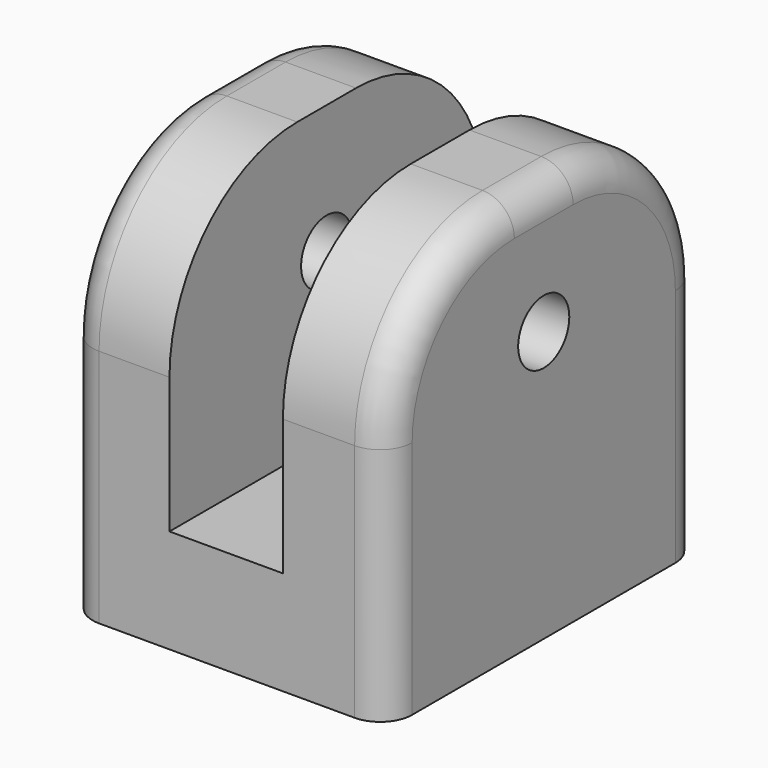
from build123d import *

# Parameters (mm, degrees)
F0_W     = 20
F0_H     = 24.5975396182
F1_DEPTH = 25
F2_W     = 7.1
F2_H     = 19.9254054902
F3_DEPTH = 12.5
F4_R     = 2
F5_DEPTH = 20.001
F6_R     = 10
F7_R     = 2
F8_R     = 2


with BuildPart() as f1:
    # F0 (on Top) → F1 (new body)
    with BuildSketch(Plane.XY):
        Rectangle(F0_W, F0_H)
    extrude(amount=F1_DEPTH)

    # F2 (on Front) → F3 (cut, symmetric)
    with BuildSketch(Plane.XZ):
        with Locations((-0.04, 16.4627027451)):
            Rectangle(F2_W, F2_H)
    extrude(amount=F3_DEPTH, both=True, mode=Mode.SUBTRACT)

    # F4 (on face) → F5 (cut, through all)
    with BuildSketch(Plane.YZ.offset(10)):
        with Locations((0, 16.9262466765)):
            Circle(F4_R)
    extrude(amount=-F5_DEPTH, mode=Mode.SUBTRACT)

    # F6
    f6_edges = [f1.edges().sort_by_distance(p)[0] for p in [
        (-6.795, -12.29877, 25),
        (6.755, -12.29877, 25),
        (6.755, 12.29877, 25),
        (-6.795, 12.29877, 25),
    ]]
    fillet(f6_edges, radius=F6_R)

    # F7
    f7_edges = [f1.edges().sort_by_distance(p)[0] for p in [
        (10, -9.369838, 22.071068),
        (10, 0, 25),
    ]]
    fillet(f7_edges, radius=F7_R)

    # F8
    f8_edges = [f1.edges().sort_by_distance(p)[0] for p in [
        (-10, 9.369838, 22.071068),
    ]]
    fillet(f8_edges, radius=F8_R)


solid = f1.part
